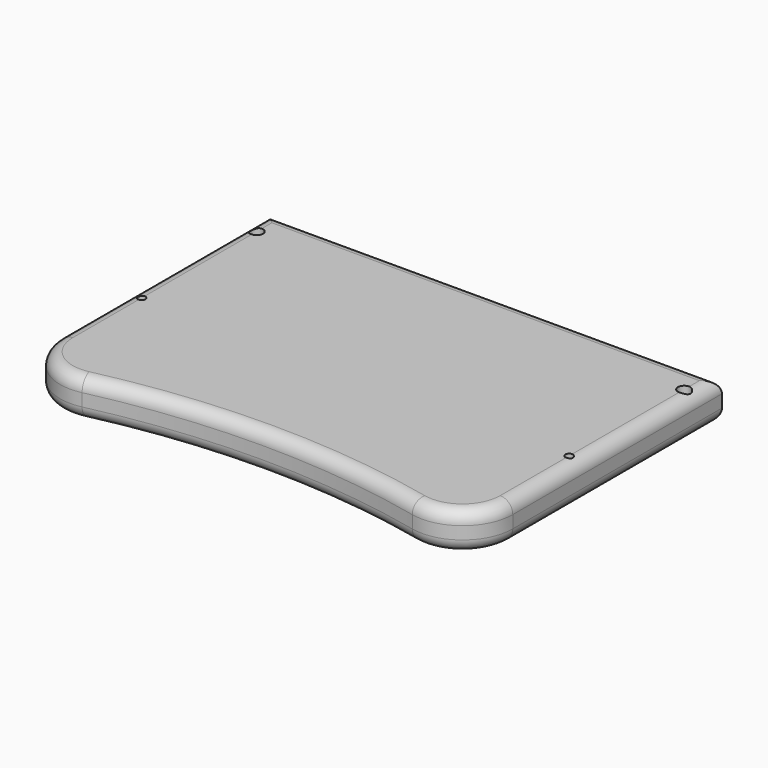
from build123d import *

# Parameters (mm, degrees)
F0_R         = 1.5
F0_R_2       = 2.5
F1_DEPTH     = 15
F2_T1_DEPTH  = 116.4597183962
F2_T3_DEPTH  = 205
F2_T6_ANGLE  = 102.5879293722
F2_T8_ANGLE  = 25.1758587444
F2_T10_ANGLE = 102.5879293722
F3_T1_DEPTH  = 205
F3_T3_DEPTH  = 116.4597183962
F3_T6_ANGLE  = 102.5879293722
F3_T8_ANGLE  = 25.1758587444
F3_T10_ANGLE = 102.5879293722


# Not quite as in the source:
# - a fillet or chamfer that OpenCascade refuses, or shapes differently, is made with other operations: its cross-section is extruded or revolved along the edge and cut away or added


with BuildPart() as f1:
    # F0 (on Top) → F1 (new body)
    with BuildSketch(Plane.XY):
        with BuildLine():
            Line((90, 69.696), (-90, 69.696))
            Line((-90, 69.696), (-90, -34.2637183962))
            ThreePointArc((-90, -34.2637183962), (-82.5064972072, -49.8710092439), (-65.6412472394, -53.7829723362))
            ThreePointArc((-65.6412472394, -53.7829723362), (0, -46.5431097607), (65.6412472394, -53.7829723362))
            ThreePointArc((65.6412472394, -53.7829723362), (82.5064972072, -49.8710092439), (90, -34.2637183962))
            Line((90, -34.2637183962), (90, 69.696))
        make_face()
        with Locations((-85, 0)):
            Circle(F0_R, mode=Mode.SUBTRACT)
        with Locations((85, 0)):
            Circle(F0_R, mode=Mode.SUBTRACT)
        with Locations((-85, 57.196)):
            Circle(F0_R_2, mode=Mode.SUBTRACT)
        with Locations((85, 57.196)):
            Circle(F0_R_2, mode=Mode.SUBTRACT)
    extrude(amount=F1_DEPTH)

    # F2: fillet of radius 5 on 2 edges, made by hand

    # F2_s2 → F2_t1 (cut)
    with BuildSketch(Plane.XZ.offset(-82.196)):
        with BuildLine():
            ThreePointArc((-90, 10), (-88.5355339059, 13.5355339059), (-85, 15))
            Line((-85, 15), (-90, 15))
            Line((-90, 15), (-90, 10))
        make_face()
        with BuildLine():
            ThreePointArc((90, 10), (88.5355339059, 13.5355339059), (85, 15))
            Line((85, 15), (90, 15))
            Line((90, 15), (90, 10))
        make_face()
    extrude(amount=F2_T1_DEPTH, mode=Mode.SUBTRACT)

    # F2_s4 → F2_t3 (cut)
    with BuildSketch(Plane.YZ.offset(-102.5)):
        with BuildLine():
            ThreePointArc((69.696, 10), (68.2315339059, 13.5355339059), (64.696, 15))
            Line((64.696, 15), (69.696, 15))
            Line((69.696, 15), (69.696, 10))
        make_face()
    extrude(amount=F2_T3_DEPTH, mode=Mode.SUBTRACT)

    # F2_s5 → F2_t6 (revolve, cut)
    with BuildSketch(Plane.XZ.offset(34.2637183962)):
        with BuildLine():
            ThreePointArc((-90, 10), (-88.5355339059, 13.5355339059), (-85, 15))
            Line((-85, 15), (-90, 15))
            Line((-90, 15), (-90, 10))
        make_face()
    revolve(axis=Axis((-70, -34.2637183962, 15), (0, 0, 1)), revolution_arc=F2_T6_ANGLE, mode=Mode.SUBTRACT)

    # F2_s7 → F2_t8 (revolve, cut)
    with BuildSketch(Plane(origin=(-73.9630818252, -16.5163478111, 0), x_dir=(0, 0, 1), z_dir=(-0.975962697, -0.217937638, 0))):
        with BuildLine():
            ThreePointArc((10, -38.1844763532), (13.5355339059, -36.7200102591), (15, -33.1844763532))
            Line((15, -33.1844763532), (15, -38.1844763532))
            Line((15, -38.1844763532), (10, -38.1844763532))
        make_face()
    revolve(axis=Axis((0, -347.7359089185, 15), (0, 0, -1)), revolution_arc=F2_T8_ANGLE, mode=Mode.SUBTRACT)

    # F2_s9 → F2_t10 (revolve, cut)
    with BuildSketch(Plane(origin=(73.9630818252, -16.5163478111, 0), x_dir=(0, 0, 1), z_dir=(-0.975962697, 0.217937638, 0))):
        with BuildLine():
            ThreePointArc((10, -38.1844763532), (13.5355339059, -36.7200102591), (15, -33.1844763532))
            Line((15, -33.1844763532), (15, -38.1844763532))
            Line((15, -38.1844763532), (10, -38.1844763532))
        make_face()
    revolve(axis=Axis((70, -34.2637183962, 15), (0, 0, 1)), revolution_arc=F2_T10_ANGLE, mode=Mode.SUBTRACT)

    # F3: fillet of radius 5 on 2 edges, made by hand

    # F3_s2 → F3_t1 (cut)
    with BuildSketch(Plane.YZ.offset(-102.5)):
        with BuildLine():
            ThreePointArc((64.696, 0), (68.2315339059, 1.4644660941), (69.696, 5))
            Line((69.696, 5), (69.696, 0))
            Line((69.696, 0), (64.696, 0))
        make_face()
    extrude(amount=F3_T1_DEPTH, mode=Mode.SUBTRACT)

    # F3_s4 → F3_t3 (cut)
    with BuildSketch(Plane.XZ.offset(-82.196)):
        with BuildLine():
            ThreePointArc((-85, 0), (-88.5355339059, 1.4644660941), (-90, 5))
            Line((-90, 5), (-90, 0))
            Line((-90, 0), (-85, 0))
        make_face()
        with BuildLine():
            ThreePointArc((85, 0), (88.5355339059, 1.4644660941), (90, 5))
            Line((90, 5), (90, 0))
            Line((90, 0), (85, 0))
        make_face()
    extrude(amount=F3_T3_DEPTH, mode=Mode.SUBTRACT)

    # F3_s5 → F3_t6 (revolve, cut)
    with BuildSketch(Plane.XZ.offset(34.2637183962)):
        with BuildLine():
            ThreePointArc((-85, 0), (-88.5355339059, 1.4644660941), (-90, 5))
            Line((-90, 5), (-90, 0))
            Line((-90, 0), (-85, 0))
        make_face()
    revolve(axis=Axis((-70, -34.2637183962, 0), (0, 0, 1)), revolution_arc=F3_T6_ANGLE, mode=Mode.SUBTRACT)

    # F3_s7 → F3_t8 (revolve, cut)
    with BuildSketch(Plane(origin=(-73.9630818252, -16.5163478111, 0), x_dir=(0, 0, 1), z_dir=(-0.975962697, -0.217937638, 0))):
        with BuildLine():
            ThreePointArc((0, -33.1844763532), (1.4644660941, -36.7200102591), (5, -38.1844763532))
            Line((5, -38.1844763532), (0, -38.1844763532))
            Line((0, -38.1844763532), (0, -33.1844763532))
        make_face()
    revolve(axis=Axis((0, -347.7359089185, 0), (0, 0, -1)), revolution_arc=F3_T8_ANGLE, mode=Mode.SUBTRACT)

    # F3_s9 → F3_t10 (revolve, cut)
    with BuildSketch(Plane(origin=(73.9630818252, -16.5163478111, 0), x_dir=(0, 0, 1), z_dir=(-0.975962697, 0.217937638, 0))):
        with BuildLine():
            ThreePointArc((5, -38.1844763532), (1.4644660941, -36.7200102591), (0, -33.1844763532))
            Line((0, -33.1844763532), (0, -38.1844763532))
            Line((0, -38.1844763532), (5, -38.1844763532))
        make_face()
    revolve(axis=Axis((70, -34.2637183962, 0), (0, 0, 1)), revolution_arc=F3_T10_ANGLE, mode=Mode.SUBTRACT)


solid = f1.part
